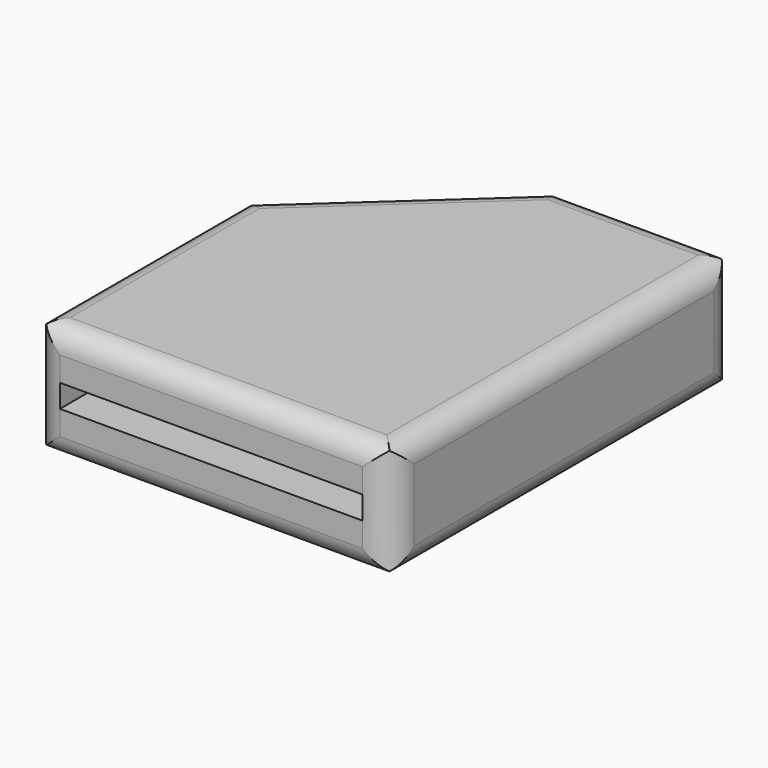
from build123d import *

# Parameters (mm, degrees)
F1_DEPTH      = 5.08
F1_DEPTH_BACK = 5.08
F2_R          = 1.905
F3_T1_DEPTH   = 19.05
F3_T3_DEPTH   = 11.9486373525
F3_T5_DEPTH   = 11.278635061
F4_W          = 26.67
F4_H          = 2.0311224633
F5_DEPTH      = 25.4


# Not quite as in the source:
# - a fillet or chamfer that OpenCascade refuses, or shapes differently, is made with other operations: its cross-section is extruded or revolved along the edge and cut away or added


with BuildPart() as f1:
    # F0 (on Top) → F1 (new body, two sides)
    with BuildSketch(Plane.XY) as f1_sk:
        Polygon((-15.875, -19.05), (15.875, -19.05), (15.875, 19.05), (0, 19.05), (-15.875, 4.5436509977), align=None)
    extrude(amount=F1_DEPTH)
    extrude(f1_sk.sketch, amount=-F1_DEPTH_BACK)

    # F2
    f2_edges = [f1.edges().sort_by_distance(p)[0] for p in [
        (-15.875, -7.253175, 5.08),
        (0, -19.05, 5.08),
        (15.875, 0, 5.08),
        (7.9375, 19.05, 5.08),
        (-7.9375, 11.796825, 5.08),
        (-15.875, -7.253175, -5.08),
        (0, -19.05, -5.08),
        (15.875, 0, -5.08),
        (7.9375, 19.05, -5.08),
        (-7.9375, 11.796825, -5.08),
    ]]
    fillet(f2_edges, radius=F2_R)

    # F3: fillet of radius 2.54 on 15 edges, made by hand

    # F3_s2 → F3_t1 (cut)
    with BuildSketch(Plane.XY.offset(-9.525)):
        with BuildLine():
            ThreePointArc((13.335, -19.05), (15.1310512242, -18.3060512242), (15.875, -16.51))
            Line((15.875, -16.51), (15.875, -19.05))
            Line((15.875, -19.05), (13.335, -19.05))
        make_face()
        with BuildLine():
            ThreePointArc((-15.875, -16.51), (-15.1310512242, -18.3060512242), (-13.335, -19.05))
            Line((-13.335, -19.05), (-15.875, -19.05))
            Line((-15.875, -19.05), (-15.875, -16.51))
        make_face()
        with BuildLine():
            ThreePointArc((13.335, 19.05), (15.1310512242, 18.3060512242), (15.875, 16.51))
            Line((15.875, 16.51), (15.875, 19.05))
            Line((15.875, 19.05), (13.335, 19.05))
        make_face()
    extrude(amount=F3_T1_DEPTH, mode=Mode.SUBTRACT)

    # F3_s4 → F3_t3 (cut)
    with BuildSketch(Plane.XY.offset(-5.9743186762)):
        with BuildLine():
            ThreePointArc((-15.875, 3.4239235272), (-15.6591819915, 4.4485103076), (-15.048403094, 5.2989834829))
            Line((-15.048403094, 5.2989834829), (-15.875, 4.5436509977))
            Line((-15.875, 4.5436509977), (-15.875, 3.4239235272))
        make_face()
    extrude(amount=F3_T3_DEPTH, mode=Mode.SUBTRACT)

    # F3_s6 → F3_t5 (cut)
    with BuildSketch(Plane.XY.offset(-5.6393175305)):
        with BuildLine():
            ThreePointArc((-0.7276760818, 18.3850599557), (0.0667744257, 18.8779371072), (0.9857270122, 19.05))
            Line((0.9857270122, 19.05), (0, 19.05))
            Line((0, 19.05), (-0.7276760818, 18.3850599557))
        make_face()
    extrude(amount=F3_T5_DEPTH, mode=Mode.SUBTRACT)

    # F4 (on face) → F5 (cut)
    with BuildSketch(Plane.XZ.offset(19.05)):
        Rectangle(F4_W, F4_H)
    extrude(amount=-F5_DEPTH, mode=Mode.SUBTRACT)


solid = f1.part
